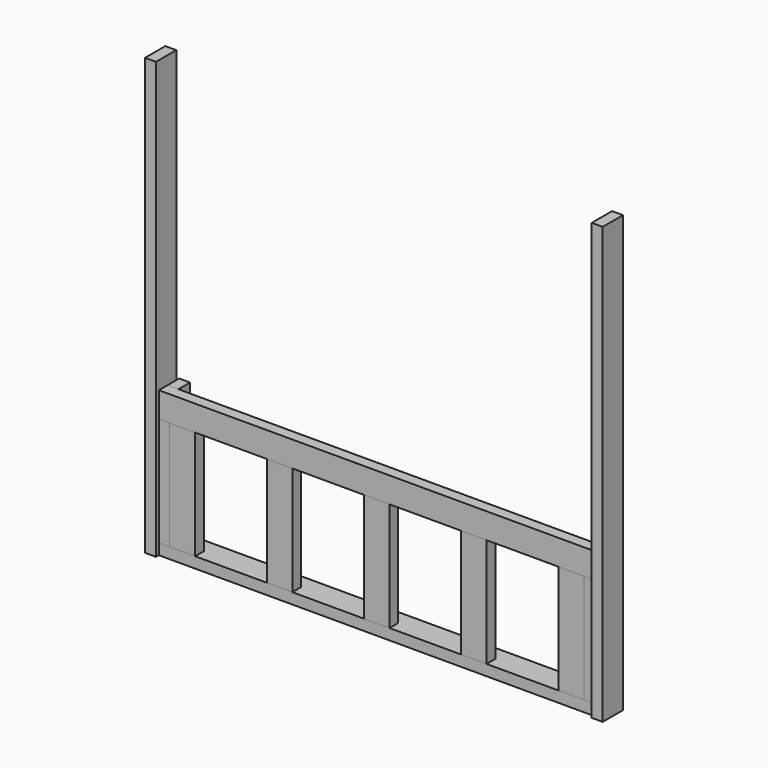
from build123d import *

# Parameters (mm, degrees)
F1_DEPTH = 1524
F0_W     = 38.1
F0_H     = 38.1
F0_W_2   = 88.9
F0_W_3   = 250.825
F2_DEPTH = 508
F3_DEPTH = 419.1
F4_DEPTH = 508
F5_DEPTH = 419.1
F6_DEPTH = 419.1
F7_DEPTH = 38.1
F8_DEPTH = 38.1


# Not quite as in the source:
# - a feature names something its author has since deleted; it is built from what else it names


with BuildPart() as f1:
    # F0 (on Top) → F1 (new body)
    with BuildSketch(Plane.XY):
        Polygon((0, -12.7), (0, 0), (0, 38.1), (0, 76.2), (-38.1, 76.2), (-38.1, -12.7), align=None)
    extrude(amount=F1_DEPTH)


with BuildPart() as f1b:
    # F0 (on Top) → F1, piece 2 (new body)
    with BuildSketch(Plane.XY):
        Polygon((1562.1, 76.2), (1524, 76.2), (1524, 38.1), (1524, 0), (1524, -12.7), (1562.1, -12.7), align=None)
    extrude(amount=F1_DEPTH)


with BuildPart() as f2:
    # F0 (on Top) → F2 (new body)
    with BuildSketch(Plane.XY):
        with Locations((19.05, 19.05)):
            Rectangle(F0_W, F0_H)
        with Locations((82.55, 19.05)):
            Rectangle(F0_W_2, F0_H)
        with Locations((252.4125, 19.05)):
            Rectangle(F0_W_3, F0_H)
        with Locations((422.275, 19.05)):
            Rectangle(F0_W_2, F0_H)
        with Locations((592.1375, 19.05)):
            Rectangle(F0_W_3, F0_H)
        with Locations((762, 19.05)):
            Rectangle(F0_W_2, F0_H)
        with Locations((931.8625, 19.05)):
            Rectangle(F0_W_3, F0_H)
        with Locations((1101.725, 19.05)):
            Rectangle(F0_W_2, F0_H)
        with Locations((1271.5875, 19.05)):
            Rectangle(F0_W_3, F0_H)
        with Locations((1441.45, 19.05)):
            Rectangle(F0_W_2, F0_H)
        with Locations((1504.95, 19.05)):
            Rectangle(F0_W, F0_H)
    extrude(amount=F2_DEPTH)

    # F0 (on Top) → F3 (cut)
    with BuildSketch(Plane.XY):
        with Locations((19.05, 19.05)):
            Rectangle(F0_W, F0_H)
        with Locations((82.55, 19.05)):
            Rectangle(F0_W_2, F0_H)
        with Locations((252.4125, 19.05)):
            Rectangle(F0_W_3, F0_H)
        with Locations((422.275, 19.05)):
            Rectangle(F0_W_2, F0_H)
        with Locations((592.1375, 19.05)):
            Rectangle(F0_W_3, F0_H)
        with Locations((762, 19.05)):
            Rectangle(F0_W_2, F0_H)
        with Locations((931.8625, 19.05)):
            Rectangle(F0_W_3, F0_H)
        with Locations((1101.725, 19.05)):
            Rectangle(F0_W_2, F0_H)
        with Locations((1271.5875, 19.05)):
            Rectangle(F0_W_3, F0_H)
        with Locations((1441.45, 19.05)):
            Rectangle(F0_W_2, F0_H)
        with Locations((1504.95, 19.05)):
            Rectangle(F0_W, F0_H)
    extrude(amount=F3_DEPTH, mode=Mode.SUBTRACT)


with BuildPart() as f4:
    # F0 (on Top) → F4 (new body, through all)
    with BuildSketch(Plane.XY):
        Polygon((0, 76.2), (0, 38.1), (38.1, 38.1), (38.1, 88.9), (0, 88.9), align=None)
    extrude(amount=F4_DEPTH)

    # F0 (on Top) → F5 (join, through all)
    with BuildSketch(Plane.XY):
        with Locations((19.05, 19.05)):
            Rectangle(F0_W, F0_H)
    extrude(amount=F5_DEPTH)


with BuildPart() as f4b:
    # F0 (on Top) → F4, piece 2 (new body, through all)
    with BuildSketch(Plane.XY):
        Polygon((1524, 88.9), (1485.9, 88.9), (1485.9, 38.1), (1524, 38.1), (1524, 76.2), align=None)
    extrude(amount=F4_DEPTH)

    # F0 (on Top) → F5, piece 2 (join, through all)
    with BuildSketch(Plane.XY):
        with Locations((1504.95, 19.05)):
            Rectangle(F0_W, F0_H)
    extrude(amount=F5_DEPTH)


with BuildPart() as f6:
    # F0 (on Top) → F6 (new body, through all)
    with BuildSketch(Plane.XY):
        with Locations((82.55, 19.05)):
            Rectangle(F0_W_2, F0_H)
    extrude(amount=F6_DEPTH)


with BuildPart() as f6b:
    # F0 (on Top) → F6, piece 2 (new body, through all)
    with BuildSketch(Plane.XY):
        with Locations((422.275, 19.05)):
            Rectangle(F0_W_2, F0_H)
    extrude(amount=F6_DEPTH)


with BuildPart() as f6c:
    # F0 (on Top) → F6, piece 3 (new body, through all)
    with BuildSketch(Plane.XY):
        with Locations((762, 19.05)):
            Rectangle(F0_W_2, F0_H)
    extrude(amount=F6_DEPTH)


with BuildPart() as f6d:
    # F0 (on Top) → F6, piece 4 (new body, through all)
    with BuildSketch(Plane.XY):
        with Locations((1101.725, 19.05)):
            Rectangle(F0_W_2, F0_H)
    extrude(amount=F6_DEPTH)


with BuildPart() as f6e:
    # F0 (on Top) → F6, piece 5 (new body, through all)
    with BuildSketch(Plane.XY):
        with Locations((1441.45, 19.05)):
            Rectangle(F0_W_2, F0_H)
    extrude(amount=F6_DEPTH)


with BuildPart() as f7_tool:
    # F0 (on Top) → F7 (new body)
    with BuildSketch(Plane.XY):
        Polygon((1524, 88.9), (1485.9, 88.9), (1485.9, 38.1), (1524, 38.1), (1524, 76.2), align=None)
        with Locations((1504.95, 19.05)):
            Rectangle(F0_W, F0_H)
        with Locations((1441.45, 19.05)):
            Rectangle(F0_W_2, F0_H)
        with Locations((1101.725, 19.05)):
            Rectangle(F0_W_2, F0_H)
        with Locations((762, 19.05)):
            Rectangle(F0_W_2, F0_H)
        with Locations((422.275, 19.05)):
            Rectangle(F0_W_2, F0_H)
        with Locations((82.55, 19.05)):
            Rectangle(F0_W_2, F0_H)
        with Locations((19.05, 19.05)):
            Rectangle(F0_W, F0_H)
        Polygon((0, 76.2), (0, 38.1), (38.1, 38.1), (38.1, 88.9), (0, 88.9), align=None)
    extrude(amount=F7_DEPTH)


with BuildPart() as f4_1:
    add(f4.part)

    # F7: cut by f7_tool
    add(f7_tool.part, mode=Mode.SUBTRACT)


with BuildPart() as f4b_1:
    add(f4b.part)

    # F7: cut by f7_tool
    add(f7_tool.part, mode=Mode.SUBTRACT)


with BuildPart() as f6_1:
    add(f6.part)

    # F7: cut by f7_tool
    add(f7_tool.part, mode=Mode.SUBTRACT)


with BuildPart() as f6b_1:
    add(f6b.part)

    # F7: cut by f7_tool
    add(f7_tool.part, mode=Mode.SUBTRACT)


with BuildPart() as f6c_1:
    add(f6c.part)

    # F7: cut by f7_tool
    add(f7_tool.part, mode=Mode.SUBTRACT)


with BuildPart() as f6d_1:
    add(f6d.part)

    # F7: cut by f7_tool
    add(f7_tool.part, mode=Mode.SUBTRACT)


with BuildPart() as f6e_1:
    add(f6e.part)

    # F7: cut by f7_tool
    add(f7_tool.part, mode=Mode.SUBTRACT)


with BuildPart() as f8:
    # F0 (on Top) → F8 (new body)
    with BuildSketch(Plane.XY):
        Polygon((1524, 88.9), (1485.9, 88.9), (1485.9, 38.1), (1524, 38.1), (1524, 76.2), align=None)
        with Locations((1504.95, 19.05)):
            Rectangle(F0_W, F0_H)
        with Locations((1441.45, 19.05)):
            Rectangle(F0_W_2, F0_H)
        Polygon((38.1, 88.9), (38.1, 38.1), (127, 38.1), (377.825, 38.1), (466.725, 38.1), (717.55, 38.1), (806.45, 38.1), (1057.275, 38.1), (1146.175, 38.1), (1397, 38.1), (1485.9, 38.1), (1485.9, 88.9), align=None)
        with Locations((1271.5875, 19.05)):
            Rectangle(F0_W_3, F0_H)
        with Locations((1101.725, 19.05)):
            Rectangle(F0_W_2, F0_H)
        with Locations((931.8625, 19.05)):
            Rectangle(F0_W_3, F0_H)
        with Locations((762, 19.05)):
            Rectangle(F0_W_2, F0_H)
        with Locations((592.1375, 19.05)):
            Rectangle(F0_W_3, F0_H)
        with Locations((422.275, 19.05)):
            Rectangle(F0_W_2, F0_H)
        with Locations((252.4125, 19.05)):
            Rectangle(F0_W_3, F0_H)
        with Locations((82.55, 19.05)):
            Rectangle(F0_W_2, F0_H)
        Polygon((0, 76.2), (0, 38.1), (38.1, 38.1), (38.1, 88.9), (0, 88.9), align=None)
        with Locations((19.05, 19.05)):
            Rectangle(F0_W, F0_H)
    extrude(amount=F8_DEPTH)


solid = Compound([f1.part, f1b.part, f2.part, f4_1.part, f4b_1.part, f6_1.part, f6b_1.part, f6c_1.part, f6d_1.part, f6e_1.part, f8.part])
